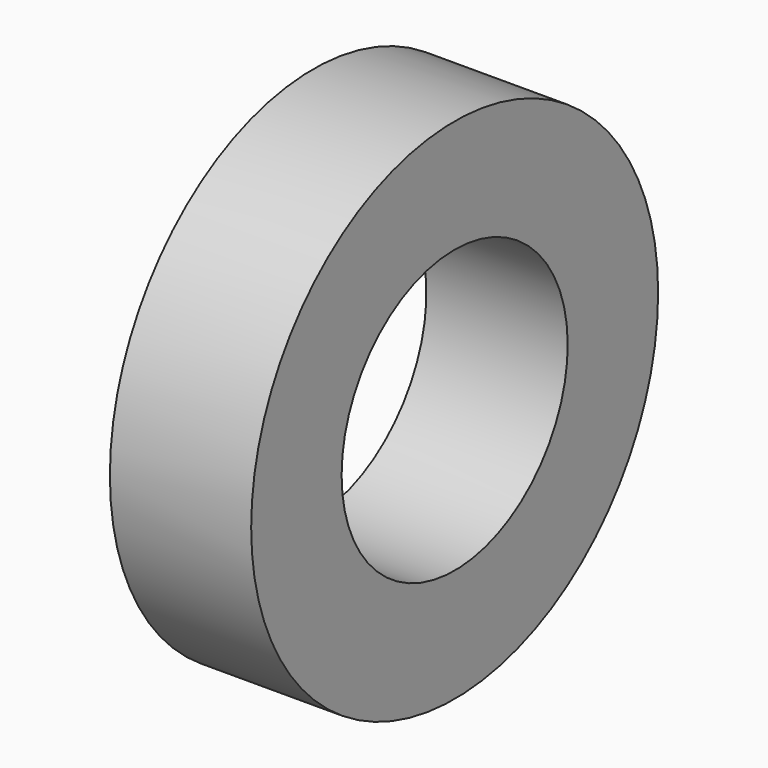
from build123d import *

# Parameters (mm, degrees)
F0_W      = 63.5
F0_H      = 63.5
F0_W_2    = 50.8
F0_H_2    = 50.8
F1_DEPTH  = 165.1
F3_R      = 6.35
F4_DEPTH  = 25.4
F6_DEPTH  = 25.4
F7_R      = 6.35
F8_DEPTH  = 63.501
F9_W      = 145.7979530096
F9_H      = 377.9422044754
F9_W_2    = 50.8
F9_H_2    = 292.1
F10_DEPTH = 63.5
F11_W     = 97.6704657078
F11_H     = 338.8985395432
F12_DEPTH = 57.151
F13_R     = 11.43
F13_R_2   = 6.35
F14_DEPTH = 6.35
F15_W     = 170.8157360554
F15_H     = 347.1174836159
F16_DEPTH = 25.4


# Not quite as in the source:
# - ends of sketch curves that miss each other by under 0.0002 mm in the source are joined


with BuildPart() as f1:
    # F0 (on Top) → F1 (new body, symmetric)
    with BuildSketch(Plane.XY):
        Rectangle(F0_W, F0_H)
        Rectangle(F0_W_2, F0_H_2, mode=Mode.SUBTRACT)
    extrude(amount=F1_DEPTH, both=True)

    # F3 (on face) → F4 (cut)
    with BuildSketch(Plane.YZ.offset(31.75)):
        with Locations((0, 146.05)):
            Circle(F3_R)
        with BuildLine():
            ThreePointArc((10.1385245046, 129.1766616857), (14.6288058895, 132.8781640138), (17.8406687878, 137.7307595176))
            ThreePointArc((17.8406687878, 137.7307595176), (19.4934269332, 143.3103775076), (19.4426449846, 149.1294124443))
            ThreePointArc((19.4426449846, 149.1294124443), (15.0835370951, 152.2964897102), (11.9164598293, 147.9373818207))
            ThreePointArc((11.9164598293, 147.9373818207), (11.9475842494, 144.3708765369), (10.9346034506, 140.9511106721))
            ThreePointArc((10.9346034506, 140.9511106721), (8.9660423194, 137.9769392343), (6.2139343738, 135.708276517))
            ThreePointArc((6.2139343738, 135.708276517), (4.9104220235, 130.4801740359), (10.1385245046, 129.1766616857))
        make_face()
        with BuildLine():
            ThreePointArc((-10.1385245046, 129.1766616857), (-4.9104220235, 130.4801740359), (-6.2139343738, 135.708276517))
            ThreePointArc((-6.2139343738, 135.708276517), (-8.9660423194, 137.9769392343), (-10.9346034506, 140.9511106721))
            ThreePointArc((-10.9346034506, 140.9511106721), (-11.9475842494, 144.3708765369), (-11.9164598293, 147.9373818207))
            ThreePointArc((-11.9164598293, 147.9373818207), (-15.0835370951, 152.2964897102), (-19.4426449846, 149.1294124443))
            ThreePointArc((-19.4426449846, 149.1294124443), (-19.4934269332, 143.3103775076), (-17.8406687878, 137.7307595176))
            ThreePointArc((-17.8406687878, 137.7307595176), (-14.6288058895, 132.8781640138), (-10.1385245046, 129.1766616857))
        make_face()
    extrude(amount=-F4_DEPTH, mode=Mode.SUBTRACT)

    # F5 (on face) → F6 (cut)
    with BuildSketch(Plane(origin=(-31.75, 0, 0), x_dir=(0, -1, 0), z_dir=(-1, 0, 0))):
        with BuildLine():
            ThreePointArc((-3.0785410886, 140.4961648597), (3.2228686048, 140.5786548312), (6.35, 146.05))
            ThreePointArc((6.35, 146.05), (-3.2228686048, 151.5213451688), (-3.0785410886, 140.4961648597))
        make_face()
        with BuildLine():
            ThreePointArc((-5.7913527214, 132.1654121492), (-6.0549491708, 133.1322727306), (-6.7727903948, 133.8315626913))
            ThreePointArc((-6.7727903948, 133.8315626913), (-9.3377562721, 131.1985515677), (-5.7913527214, 132.1654121492))
        make_face()
        with BuildLine():
            ThreePointArc((3.1226517792, 134.3961049058), (0.4285749428, 129.7298269458), (5.0948529028, 127.0357501095))
            ThreePointArc((5.0948529028, 127.0357501095), (17.8406687878, 137.7307595176), (17.8406687878, 154.3692404824))
            ThreePointArc((17.8406687878, 154.3692404824), (12.777460542, 156.2120975737), (10.9346034506, 151.1488893279))
            ThreePointArc((10.9346034506, 151.1488893279), (10.9346034506, 140.9511106721), (3.1226517792, 134.3961049058))
        make_face()
    extrude(amount=-F6_DEPTH, mode=Mode.SUBTRACT)

    # F7 (on face) → F8 (cut, through all)
    with BuildSketch(Plane.YZ.offset(31.75)):
        with BuildLine():
            ThreePointArc((-8.89, 107.949999693), (-15.239999693, 101.6), (-8.89, 95.250000307))
            ThreePointArc((-8.89, 95.250000307), (3.81, 82.55), (-8.89, 69.85))
            ThreePointArc((-8.89, 69.85), (-15.239999693, 63.5), (-8.89, 57.150000307))
            ThreePointArc((-8.89, 57.150000307), (16.509999693, 82.55), (-8.89, 107.949999693))
        make_face()
        with BuildLine():
            ThreePointArc((8.89, 3.07e-07), (15.239999693, 6.35), (8.89, 12.699999693))
            ThreePointArc((8.89, 12.699999693), (-3.81, 25.4), (8.89, 38.1))
            ThreePointArc((8.89, 38.1), (15.24, 44.45), (8.89, 50.8))
            ThreePointArc((8.89, 50.8), (-16.509999693, 25.4), (8.89, 3.07e-07))
        make_face()
        with BuildLine():
            ThreePointArc((-8.89, -6.350000307), (-15.239999693, -12.7), (-8.89, -19.049999693))
            ThreePointArc((-8.89, -19.049999693), (3.81, -31.75), (-8.89, -44.45))
            ThreePointArc((-8.89, -44.45), (-15.239999693, -50.8), (-8.89, -57.149999693))
            ThreePointArc((-8.89, -57.149999693), (16.509999693, -31.75), (-8.89, -6.350000307))
        make_face()
        with BuildLine():
            ThreePointArc((8.89, -114.299999693), (15.239999693, -107.95), (8.89, -101.600000307))
            ThreePointArc((8.89, -101.600000307), (-3.81, -88.9), (8.89, -76.2))
            ThreePointArc((8.89, -76.2), (15.24, -69.85), (8.89, -63.5))
            ThreePointArc((8.89, -63.5), (-16.509999693, -88.9), (8.89, -114.299999693))
        make_face()
        with Locations((-8.89, 82.55)):
            Circle(F7_R)
        with Locations((8.89, 25.4)):
            Circle(F7_R)
        with Locations((8.89, -88.9)):
            Circle(F7_R)
        with Locations((-8.89, -31.75)):
            Circle(F7_R)
    extrude(amount=-F8_DEPTH, mode=Mode.SUBTRACT)

    # F9 (on face) → F10 (cut, symmetric)
    with BuildSketch(Plane(origin=(25.4, 0, 0), x_dir=(0, -1, 0), z_dir=(-1, 0, 0))):
        Rectangle(F9_W, F9_H)
        with Locations((0, 19.05)):
            Rectangle(F9_W_2, F9_H_2, mode=Mode.SUBTRACT)
    extrude(amount=F10_DEPTH, both=True, mode=Mode.SUBTRACT)

    # F11 (on face) → F12 (cut, through all)
    with BuildSketch(Plane.YZ.offset(-25.4)):
        Rectangle(F11_W, F11_H)
    extrude(amount=F12_DEPTH, mode=Mode.SUBTRACT)

    # F13 (on face) → F14 (join)
    with BuildSketch(Plane(origin=(-31.75, 0, 0), x_dir=(0, -1, 0), z_dir=(-1, 0, 0))):
        with Locations((0, 146.05)):
            Circle(F13_R)
        with Locations((0, 146.05)):
            Circle(F13_R_2, mode=Mode.SUBTRACT)
    extrude(amount=F14_DEPTH)

    # F15 (on face) → F16 (cut)
    with BuildSketch(Plane(origin=(-31.75, 0, 0), x_dir=(0, -1, 0), z_dir=(-1, 0, 0))):
        Rectangle(F15_W, F15_H)
    extrude(amount=-F16_DEPTH, mode=Mode.SUBTRACT)


solid = f1.part
